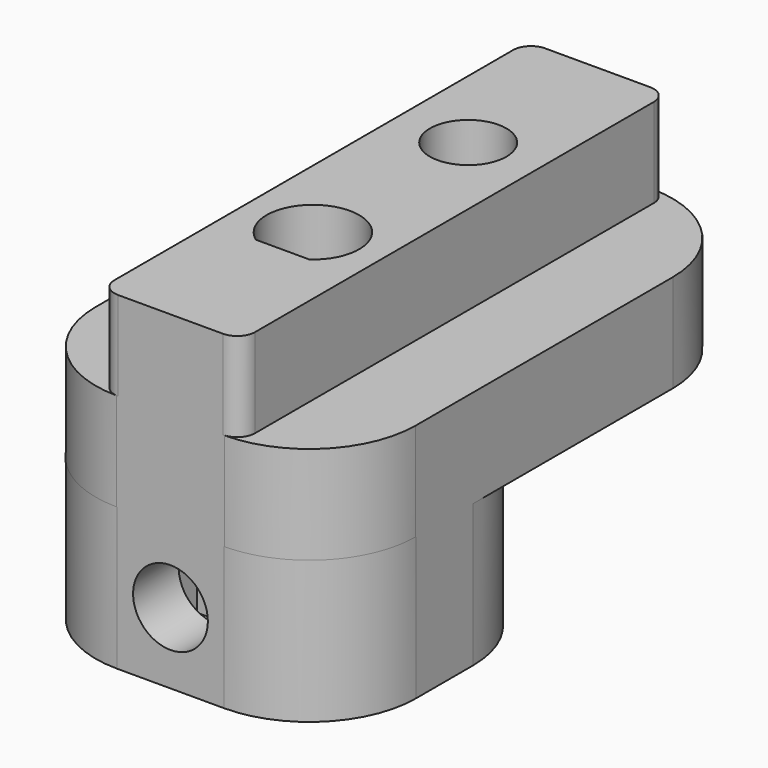
from build123d import *

# Parameters (mm, degrees)
F0_W         = 18
F0_H         = 16
F0_W_2       = 7.2
F0_H_2       = 3.15
F1_DEPTH     = 8
F2_R         = 6
F4_R         = 2.1
F5_DEPTH     = 10
F7_R         = 2.15
F8_DEPTH     = 5.5
F9_DEPTH     = 2.5
F10_T1_DEPTH = 35.4995000042
F12_R        = 2.15
F13_DEPTH    = 5
F14_T1_DEPTH = 7.5071501803


# Not quite as in the source:
# - a fillet or chamfer that OpenCascade refuses, or shapes differently, is made with other operations: its cross-section is extruded or revolved along the edge and cut away or added


with BuildPart() as f1:
    # F0 (on Top) → F1 (new body)
    with BuildSketch(Plane.XY):
        with Locations((0, -2)):
            Rectangle(F0_W, F0_H)
        with Locations((0, -5.225)):
            Rectangle(F0_W_2, F0_H_2, mode=Mode.SUBTRACT)
        with BuildLine():
            ThreePointArc((-1.5, -2.1236760582), (-1.1958260743, 2.3086792761), (2.6, 0))
            ThreePointArc((2.6, 0), (2.3086792761, -1.1958260743), (1.5, -2.1236760582))
            ThreePointArc((1.5, -2.1236760582), (0, -2.6), (-1.5, -2.1236760582))
        make_face(mode=Mode.SUBTRACT)
        with BuildLine():
            Line((1.5, -2.1236760582), (-1.5, -2.1236760582))
            ThreePointArc((-1.5, -2.1236760582), (0, -2.6), (1.5, -2.1236760582))
        make_face()
    extrude(amount=F1_DEPTH)

    # F2
    f2_edges = [f1.edges().sort_by_distance(p)[0] for p in [
        (9, -10, 4),
        (-9, -10, 4),
        (9, 6, 4),
        (-9, 6, 4),
    ]]
    fillet(f2_edges, radius=F2_R)

    # F4 (on offset) → F5 (cut)
    with BuildSketch(Plane.XZ.offset(10)):
        with Locations((0, 4)):
            Circle(F4_R)
    extrude(amount=-F5_DEPTH, mode=Mode.SUBTRACT)

    # F7 (on offset) → F8 (join)
    with BuildSketch(Plane.XY.offset(8)):
        Polygon((-9, 20), (-9, 0), (-9, -4), (-9, -10), (-3, -10), (3, -10), (9, -10), (9, -4), (9, 0), (9, 20), align=None)
        with BuildLine():
            ThreePointArc((-1.5, -2.1236760582), (0, 2.6), (1.5, -2.1236760582))
            Line((1.5, -2.1236760582), (-1.5, -2.1236760582))
        make_face(mode=Mode.SUBTRACT)
        with BuildLine():
            ThreePointArc((2.075, 14.5), (3.5940054257, 12.9809945743), (4.15, 10.9059945743))
            ThreePointArc((4.15, 10.9059945743), (3.5940054257, 8.8309945743), (2.075, 7.3119891486))
            ThreePointArc((2.075, 7.3119891486), (0, 6.7559945743), (-2.075, 7.3119891486))
            ThreePointArc((-2.075, 7.3119891486), (-3.5940054257, 8.8309945743), (-4.15, 10.9059945743))
            ThreePointArc((-4.15, 10.9059945743), (-3.5940054257, 12.9809945743), (-2.075, 14.5))
            ThreePointArc((-2.075, 14.5), (0, 15.0559945743), (2.075, 14.5))
        make_face(mode=Mode.SUBTRACT)
        with BuildLine():
            ThreePointArc((-4.15, 10.9059945743), (-3.5940054257, 8.8309945743), (-2.075, 7.3119891486))
            Line((-2.075, 7.3119891486), (-4.15, 10.9059945743))
        make_face()
        with BuildLine():
            Line((-4.15, 10.9059945743), (-2.075, 14.5))
            ThreePointArc((-2.075, 14.5), (-3.5940054257, 12.9809945743), (-4.15, 10.9059945743))
        make_face()
        with BuildLine():
            Line((-2.075, 14.5), (2.075, 14.5))
            ThreePointArc((2.075, 14.5), (0, 15.0559945743), (-2.075, 14.5))
        make_face()
        with BuildLine():
            Line((2.075, 14.5), (4.15, 10.9059945743))
            ThreePointArc((4.15, 10.9059945743), (3.5940054257, 12.9809945743), (2.075, 14.5))
        make_face()
        with BuildLine():
            ThreePointArc((2.075, 7.3119891486), (3.5940054257, 8.8309945743), (4.15, 10.9059945743))
            Line((4.15, 10.9059945743), (2.075, 7.3119891486))
        make_face()
        with BuildLine():
            ThreePointArc((-2.075, 7.3119891486), (0, 6.7559945743), (2.075, 7.3119891486))
            Line((2.075, 7.3119891486), (-2.075, 7.3119891486))
        make_face()
        Polygon((2.075, 7.3119891486), (4.15, 10.9059945743), (2.075, 14.5), (-2.075, 14.5), (-4.15, 10.9059945743), (-2.075, 7.3119891486), align=None)
        with Locations((0, 10.9059945743)):
            Circle(F7_R, mode=Mode.SUBTRACT)
    extrude(amount=F8_DEPTH)

    # F7 (on offset) → F9 (cut)
    with BuildSketch(Plane.XY.offset(8)):
        Polygon((2.075, 7.3119891486), (4.15, 10.9059945743), (2.075, 14.5), (-2.075, 14.5), (-4.15, 10.9059945743), (-2.075, 7.3119891486), align=None)
        with Locations((0, 10.9059945743)):
            Circle(F7_R, mode=Mode.SUBTRACT)
    extrude(amount=F9_DEPTH, mode=Mode.SUBTRACT)

    # F10: fillet of radius 6 on 4 edges, made by hand

    # F10_s2 → F10_t1 (cut)
    with BuildSketch(Plane.XY.offset(-6.9997500021)):
        with BuildLine():
            ThreePointArc((-9.0001, -4.0001), (-7.2427406871, -8.2427406871), (-3.0001, -10.0001))
            Line((-3.0001, -10.0001), (-3.0001, -10.1201))
            ThreePointArc((-3.0001, -10.1201), (-6.00005, -10.12), (-9, -10.12))
            Line((-9, -10.12), (-9.12, -10))
            ThreePointArc((-9.12, -10), (-9.12, -7.00005), (-9.1201, -4.0001))
            Line((-9.1201, -4.0001), (-9.0001, -4.0001))
        make_face()
        with BuildLine():
            ThreePointArc((9.0001, -4.0001), (7.2427406871, -8.2427406871), (3.0001, -10.0001))
            Line((3.0001, -10.0001), (3.0001, -10.1201))
            ThreePointArc((3.0001, -10.1201), (6.00005, -10.12), (9, -10.12))
            Line((9, -10.12), (9.12, -10))
            ThreePointArc((9.12, -10), (9.12, -7.00005), (9.1201, -4.0001))
            Line((9.1201, -4.0001), (9.0001, -4.0001))
        make_face()
        with BuildLine():
            ThreePointArc((9.0001, 14.0001), (7.2427406871, 18.2427406871), (3.0001, 20.0001))
            Line((3.0001, 20.0001), (3.0001, 20.1201))
            ThreePointArc((3.0001, 20.1201), (6.00005, 20.12), (9, 20.12))
            Line((9, 20.12), (9.12, 20))
            ThreePointArc((9.12, 20), (9.12, 17.00005), (9.1201, 14.0001))
            Line((9.1201, 14.0001), (9.0001, 14.0001))
        make_face()
        with BuildLine():
            ThreePointArc((-9.0001, 14.0001), (-7.2427406871, 18.2427406871), (-3.0001, 20.0001))
            Line((-3.0001, 20.0001), (-3.0001, 20.1201))
            ThreePointArc((-3.0001, 20.1201), (-6.00005, 20.12), (-9, 20.12))
            Line((-9, 20.12), (-9.12, 20))
            ThreePointArc((-9.12, 20), (-9.12, 17.00005), (-9.1201, 14.0001))
            Line((-9.1201, 14.0001), (-9.0001, 14.0001))
        make_face()
    extrude(amount=F10_T1_DEPTH, mode=Mode.SUBTRACT)

    # F12 (on offset) → F13 (join)
    with BuildSketch(Plane.XY.offset(13.5)):
        with BuildLine():
            Line((-3.95, 19.9243143063), (-3.95, -9.9243143063))
            ThreePointArc((-3.95, -9.9243143063), (-3.4765050693, -9.9810486471), (-3, -10))
            Line((-3, -10), (3, -10))
            ThreePointArc((3, -10), (3.4765050693, -9.9810486471), (3.95, -9.9243143063))
            Line((3.95, -9.9243143063), (3.95, 19.9243143063))
            ThreePointArc((3.95, 19.9243143063), (3.4765050693, 19.9810486471), (3, 20))
            Line((3, 20), (-3, 20))
            ThreePointArc((-3, 20), (-3.4765050693, 19.9810486471), (-3.95, 19.9243143063))
        make_face()
        with BuildLine():
            Line((1.5, -2.1236760582), (-1.5, -2.1236760582))
            ThreePointArc((-1.5, -2.1236760582), (0, 2.6), (1.5, -2.1236760582))
        make_face(mode=Mode.SUBTRACT)
        with Locations((0, 10.9059945743)):
            Circle(F12_R, mode=Mode.SUBTRACT)
    extrude(amount=F13_DEPTH)

    # F14: fillet of radius 1 on 4 edges, made by hand

    # F14_s2 → F14_t1 (cut)
    with BuildSketch(Plane.XY.offset(13.5)):
        with BuildLine():
            ThreePointArc((3.95, -9), (3.6571067812, -9.7071067812), (2.95, -10))
            Line((2.95, -10), (2.95, -10.1))
            ThreePointArc((2.95, -10.1), (3, -10.1), (3.9658333333, -10.0230528781))
            Line((3.9658333333, -10.0230528781), (4.05, -9.9243143063))
            Line((4.05, -9.9243143063), (4.05, -9))
            Line((4.05, -9), (3.95, -9))
        make_face()
        with BuildLine():
            ThreePointArc((-2.95, -10), (-3.6571067812, -9.7071067812), (-3.95, -9))
            Line((-3.95, -9), (-4.05, -9))
            Line((-4.05, -9), (-4.05, -9.9243143063))
            Line((-4.05, -9.9243143063), (-3.9658333333, -10.0230528781))
            ThreePointArc((-3.9658333333, -10.0230528781), (-3, -10.1), (-2.95, -10.1))
            Line((-2.95, -10.1), (-2.95, -10))
        make_face()
        with BuildLine():
            ThreePointArc((2.95, 20), (3.6571067812, 19.7071067812), (3.95, 19))
            Line((3.95, 19), (4.05, 19))
            Line((4.05, 19), (4.05, 19.9243143063))
            Line((4.05, 19.9243143063), (3.9658333333, 20.0230528781))
            ThreePointArc((3.9658333333, 20.0230528781), (3, 20.1), (2.95, 20.1))
            Line((2.95, 20.1), (2.95, 20))
        make_face()
        with BuildLine():
            ThreePointArc((-2.95, 20), (-3.6571067812, 19.7071067812), (-3.95, 19))
            Line((-3.95, 19), (-4.05, 19))
            Line((-4.05, 19), (-4.05, 19.9243143063))
            Line((-4.05, 19.9243143063), (-3.9658333333, 20.0230528781))
            ThreePointArc((-3.9658333333, 20.0230528781), (-3, 20.1), (-2.95, 20.1))
            Line((-2.95, 20.1), (-2.95, 20))
        make_face()
    extrude(amount=F14_T1_DEPTH, mode=Mode.SUBTRACT)


solid = f1.part
